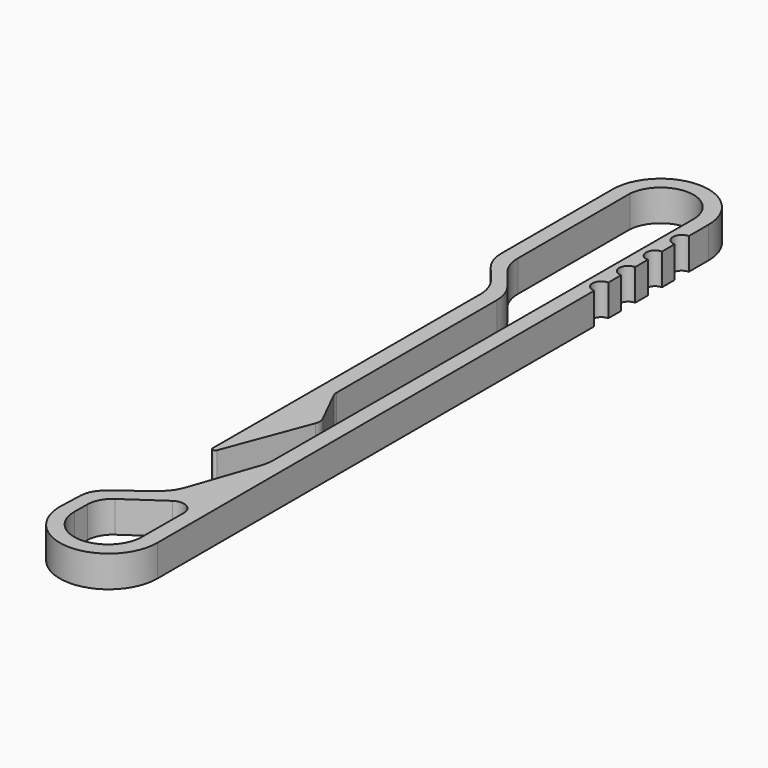
from build123d import *

# Parameters (mm, degrees)
F1_DEPTH = 2.5
F2_R     = 1
F3_R     = 0.2
F4_R     = 1
F5_R     = 3
F6_R     = 3
F7_R     = 3
F8_R     = 3
F9_R     = 2
F10_R    = 2
F11_R    = 3
F12_R    = 1


# Not quite as in the source:
# - ends of sketch curves that miss each other by under 0.0002 mm in the source are joined


with BuildPart() as f1:
    # F0 (on Top) → F1 (new body)
    with BuildSketch(Plane.XY):
        with BuildLine():
            Line((-3.7337125044, -24.7166411829), (-3.8395490403, -27.4549634883))
            ThreePointArc((-3.8395490403, -27.4549634883), (-0.0393100387, -31.4820484538), (3.9136249429, -27.6047381979))
            Line((3.9136249429, -27.6047381979), (3.9136249429, 15.7631997109))
            ThreePointArc((3.9136249429, 15.7631997109), (3.2136249429, 16.4631997109), (3.9136249429, 17.1631997109))
            Line((3.9136249429, 17.1631997109), (3.9136249429, 18.4257015441))
            ThreePointArc((3.9136249429, 18.4257015441), (3.2136249429, 19.1257015441), (3.9136249429, 19.8257015441))
            Line((3.9136249429, 19.8257015441), (3.9136249429, 21.0882033773))
            ThreePointArc((3.9136249429, 21.0882033773), (3.2136249429, 21.7882033773), (3.9136249429, 22.4882033773))
            Line((3.9136249429, 22.4882033773), (3.9136249429, 23.7507052105))
            ThreePointArc((3.9136249429, 23.7507052105), (3.2136249429, 24.4507052105), (3.9136249429, 25.1507052105))
            Line((3.9136249429, 25.1507052105), (3.9136249429, 27.1132070437))
            ThreePointArc((3.9136249429, 27.1132070437), (0.1053655494, 30.9191937737), (-3.7028938442, 27.1132070437))
            Line((-3.7028938442, 27.1132070437), (-3.7101279046, 14.9948472524))
            Line((-3.7101279046, 14.9948472524), (-1.3026787113, 12.0476867709))
            Line((-1.3026787113, 12.0476867709), (-1.3526145996, -16.6168491978))
            Line((-1.3526145996, -16.6168491978), (1.6919830966, -8.5560908617))
            Line((1.6919830966, -8.5560908617), (-0.0073911714, -5.1353744853))
            Line((-0.0073911714, -5.1353744853), (-0.0073911714, 12.04390363))
            Line((-0.0073911714, 12.04390363), (-2.5009698886, 15.147203732))
            Line((-2.5009698886, 15.147203732), (-2.5009698886, 27.3470994339))
            ThreePointArc((-2.5009698886, 27.3470994339), (0.2224335348, 29.7253272746), (2.7223778727, 27.1132070292))
            Line((2.7223778727, 27.1132070292), (2.7223883904, 27.1109336758))
            Line((2.7223883904, 27.1109336758), (2.6088146402, -14.972403604))
            Line((2.6088146402, -14.972403604), (0.3495425781, -21.5565683108))
            Line((0.3495425781, -21.5565683108), (-3.7337125044, -24.7166411829))
        make_face()
        with BuildLine():
            ThreePointArc((2.6714254586, -27.6047381979), (-0.0471437397, -30.2812376007), (-2.7139096259, -27.5531197061))
            Line((-2.7139096259, -27.5531197061), (-2.6834930082, -25.2417523976))
            Line((-2.6834930082, -25.2417523976), (2.7000635964, -21.5408525771))
            Line((2.7000635964, -21.5408525771), (2.6714254586, -27.6047381979))
        make_face(mode=Mode.SUBTRACT)
    extrude(amount=F1_DEPTH)

    # F2
    f2_edges = [f1.edges().sort_by_distance(p)[0] for p in [
        (2.700064, -21.540853, 1.25),
    ]]
    fillet(f2_edges, radius=F2_R)

    # F3
    f3_edges = [f1.edges().sort_by_distance(p)[0] for p in [
        (-1.352615, -16.616849, 1.25),
    ]]
    fillet(f3_edges, radius=F3_R)

    # F4
    f4_edges = [f1.edges().sort_by_distance(p)[0] for p in [
        (1.691983, -8.556091, 1.25),
    ]]
    fillet(f4_edges, radius=F4_R)

    # F5
    f5_edges = [f1.edges().sort_by_distance(p)[0] for p in [
        (-2.50097, 15.147204, 1.25),
    ]]
    fillet(f5_edges, radius=F5_R)

    # F6
    f6_edges = [f1.edges().sort_by_distance(p)[0] for p in [
        (-3.710128, 14.994847, 1.25),
    ]]
    fillet(f6_edges, radius=F6_R)

    # F7
    f7_edges = [f1.edges().sort_by_distance(p)[0] for p in [
        (-1.302679, 12.047687, 1.25),
    ]]
    fillet(f7_edges, radius=F7_R)

    # F8
    f8_edges = [f1.edges().sort_by_distance(p)[0] for p in [
        (-0.007391, 12.043904, 1.25),
    ]]
    fillet(f8_edges, radius=F8_R)

    # F9
    f9_edges = [f1.edges().sort_by_distance(p)[0] for p in [
        (-3.733713, -24.716641, 1.25),
    ]]
    fillet(f9_edges, radius=F9_R)

    # F10
    f10_edges = [f1.edges().sort_by_distance(p)[0] for p in [
        (-2.683493, -25.241752, 1.25),
    ]]
    fillet(f10_edges, radius=F10_R)

    # F11
    f11_edges = [f1.edges().sort_by_distance(p)[0] for p in [
        (0.349543, -21.556568, 1.25),
        (2.608815, -14.972404, 1.25),
    ]]
    fillet(f11_edges, radius=F11_R)

    # F12
    f12_edges = [f1.edges().sort_by_distance(p)[0] for p in [
        (-0.007391, -5.135374, 1.25),
    ]]
    fillet(f12_edges, radius=F12_R)


solid = f1.part
